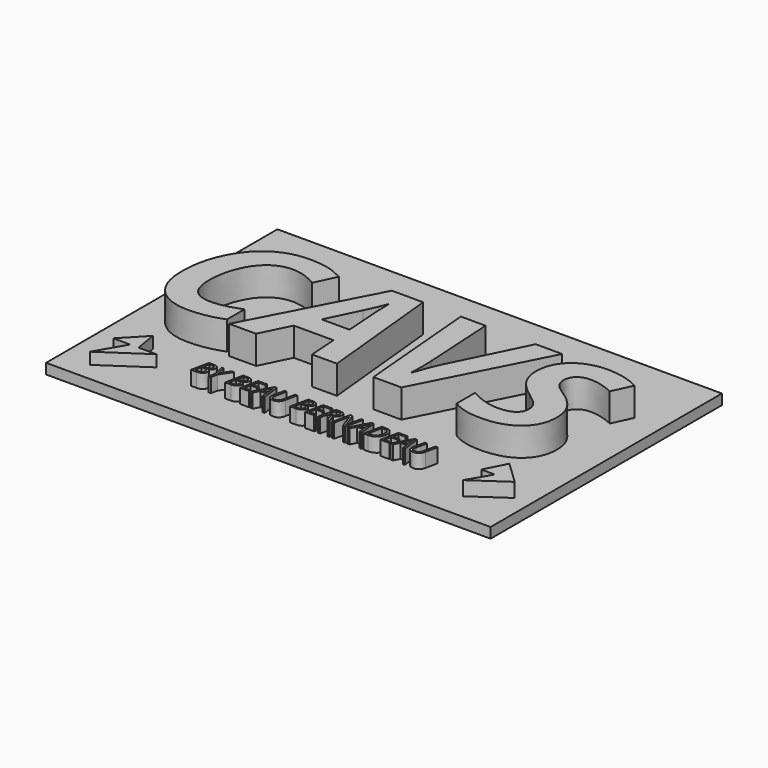
from build123d import *

# Parameters (mm, degrees)
F0_W         = 87.5685475767
F0_H         = 56.96564354
F1_DEPTH     = 2.032
F2_TEXT_SIZE = 33.8291749358
F3_DEPTH     = 5.588
F4_TEXT_SIZE = 4.9313617996
F5_DEPTH     = 2.794
F7_DEPTH     = 2.286
F9_DEPTH     = 2.794


# Not quite as in the source:
# - Text() gives the source's letters only with a copy of the font that has no kerning and outlines rounded to 1/6400 em; it was checked with that copy


with BuildPart() as f1:
    # F0 (on Top) → F1 (new body)
    with BuildSketch(Plane.XY):
        with Locations((-3.3183898777, -5.7150004432)):
            Rectangle(F0_W, F0_H)
    extrude(amount=F1_DEPTH)

    # F2 (on face) → F3 (join)
    with BuildSketch(Plane.XY.offset(2.032)):
        with Locations((-45.1890733093, -14.8437544703)):
            Text('CAVS', F2_TEXT_SIZE, font='Open Sans', font_style=FontStyle.BOLDITALIC, text_align=(TextAlign.LEFT, TextAlign.BOTTOM))
    extrude(amount=F3_DEPTH)

    # F4 (on face) → F5 (join)
    with BuildSketch(Plane.XY.offset(2.032)):
        with Locations((-25.0871432654, -26.2705665082)):
            Text('BY BEAU BERNADEAU', F4_TEXT_SIZE, font='Open Sans', font_style=FontStyle.ITALIC, text_align=(TextAlign.LEFT, TextAlign.BOTTOM))
    extrude(amount=F5_DEPTH)

    # F6 (on face) → F7 (join)
    with BuildSketch(Plane.XY.offset(2.032)):
        Polygon((-36.4100821316, -24.7957259417), (-37.1474996209, -20.37120983), (-41.3876622915, -24.7957259417), (-38.0692742765, -24.7957259417), (-41.3876622915, -30.5107254535), (-32.9073406756, -24.7957259417), align=None)
    extrude(amount=F7_DEPTH)

    # F8 (on face) → F9 (join)
    with BuildSketch(Plane.XY.offset(2.032)):
        Polygon((37.3131595552, -24.3296603032), (32.9030379653, -20.1051607728), (30.7422466756, -24.3296603032), (33.396974206, -24.3296603032), (30.7422466756, -28.8569387048), align=None)
    extrude(amount=F9_DEPTH)


solid = f1.part
